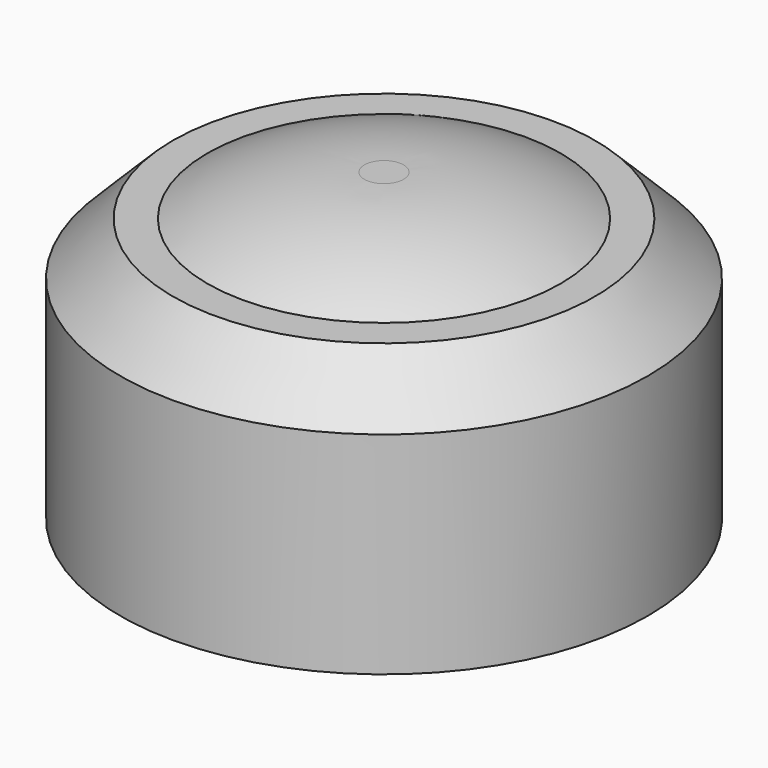
from build123d import *

# Parameters (mm, degrees)
F0_W    = 50
F0_H    = 50
F2_W    = 33.4539487958
F2_H    = 22.2039483488
F5_SIZE = 10


# Not quite as in the source:
# - a fillet or chamfer that OpenCascade refuses, or shapes differently, is made with other operations: its cross-section is extruded or revolved along the edge and cut away or added


with BuildPart() as f1:
    # F0 (on Front) → F1 (revolve)
    with BuildSketch(Plane.XZ):
        with Locations((-25, 25)):
            Rectangle(F0_W, F0_H)
    revolve(axis=Axis((0, 0, 25), (0, 0, 1)))

    # F2 (on Front) → F3 (revolve)
    with BuildSketch(Plane.XZ):
        with Locations((-16.7269743979, 46.6282907873)):
            Rectangle(F2_W, F2_H)
    revolve(axis=Axis((0, 0, 50), (0, 0, -1)))

    # F4: fillet of radius 61.079603128 on 1 edges, made by hand

    # F4_s1 → F4_t2 (revolve, cut)
    with BuildSketch(Plane.XZ):
        with BuildLine():
            ThreePointArc((-33.4539487958, 50), (-19.0772136264, 55.7661180216), (-3.7122939075, 57.7302649617))
            Line((-3.7122939075, 57.7302649617), (-33.4539487958, 57.7302649617))
            Line((-33.4539487958, 57.7302649617), (-33.4539487958, 50))
        make_face()
    revolve(axis=Axis((0, 0, 57.7302649617), (0, 0, -1)), mode=Mode.SUBTRACT)

    # F5
    f5_edges = [f1.edges().sort_by_distance(p)[0] for p in [
        (50, 0, 50),
    ]]
    chamfer(f5_edges, length=F5_SIZE)


solid = f1.part
